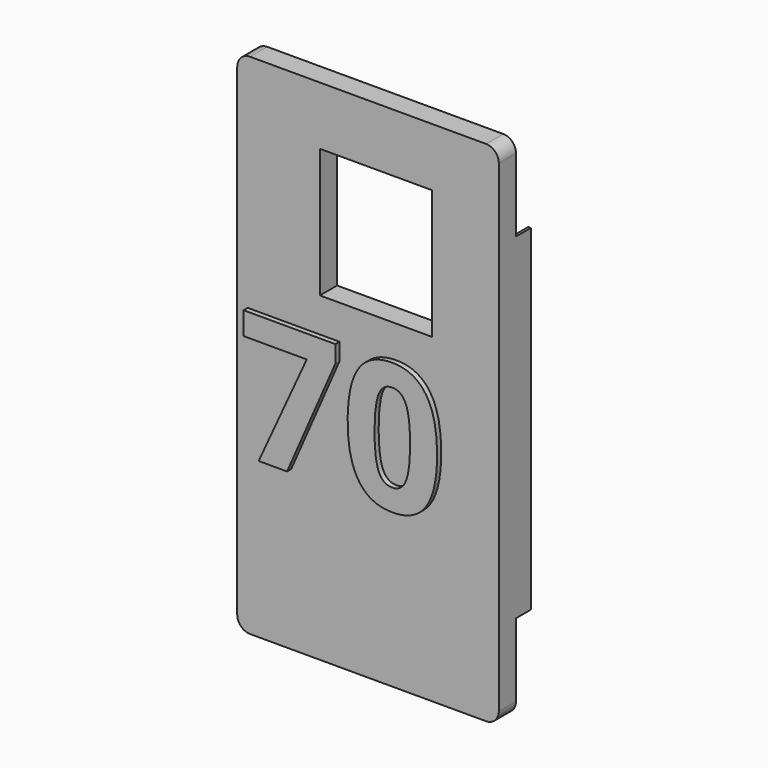
from build123d import *

# Parameters (mm, degrees)
F0_W         = 33.02
F0_H         = 38.1
F1_DEPTH     = 3.175
F2_W         = 5.4451269098
F2_H         = 99.2
F3_DEPTH     = 0.762
F4_W         = 5.4356
F4_H         = 99.2
F5_DEPTH     = 0.762
F6_TEXT_SIZE = 52.9166666667
F7_DEPTH     = 1.524


# Not quite as in the source:
# - Text() gives the source's letters only with a copy of the font that has no kerning and outlines rounded to 1/6400 em; it was checked with that copy


with BuildPart() as f1:
    # F0 (on Front) → F1 (new body, symmetric)
    with BuildSketch(Plane.XZ):
        with BuildLine():
            Line((54.6462944537, 103.9608598232), (-14.9537055463, 103.9608598232))
            ThreePointArc((-14.9537055463, 103.9608598232), (-17.6407113148, 102.8478655917), (-18.7537055463, 100.1608598232))
            Line((-18.7537055463, 100.1608598232), (-18.7537055463, -42.2391401768))
            ThreePointArc((-18.7537055463, -42.2391401768), (-17.6407113148, -44.9261459453), (-14.9537055463, -46.0391401768))
            Line((-14.9537055463, -46.0391401768), (54.6462944537, -46.0391401768))
            ThreePointArc((54.6462944537, -46.0391401768), (57.3333002222, -44.9261459453), (58.4462944537, -42.2391401768))
            Line((58.4462944537, -42.2391401768), (58.4462944537, 100.1608598232))
            ThreePointArc((58.4462944537, 100.1608598232), (57.3333002222, 102.8478655917), (54.6462944537, 103.9608598232))
        make_face()
        with Locations((22.1534632279, 67.6941627145)):
            Rectangle(F0_W, F0_H, mode=Mode.SUBTRACT)
    extrude(amount=F1_DEPTH, both=True)

    # F2 (on face) → F3 (join)
    with BuildSketch(Plane(origin=(-18.7537055463, 0, 0), x_dir=(0, -1, 0), z_dir=(-1, 0, 0))):
        with Locations((-5.8975634549, 28.9608598232)):
            Rectangle(F2_W, F2_H)
    extrude(amount=-F3_DEPTH)

    # F4 (on face) → F5 (join)
    with BuildSketch(Plane.YZ.offset(58.4462944537)):
        with Locations((5.8928, 28.9608598232)):
            Rectangle(F4_W, F4_H)
    extrude(amount=-F5_DEPTH)

    # F6 (on face) → F7 (join)
    with BuildSketch(Plane.XZ.offset(3.175)):
        with Locations((-17.0700305092, 0.7648444561)):
            Text('70', F6_TEXT_SIZE, font='Open Sans', font_style=FontStyle.BOLD, text_align=(TextAlign.LEFT, TextAlign.BOTTOM))
    extrude(amount=F7_DEPTH)


solid = f1.part
